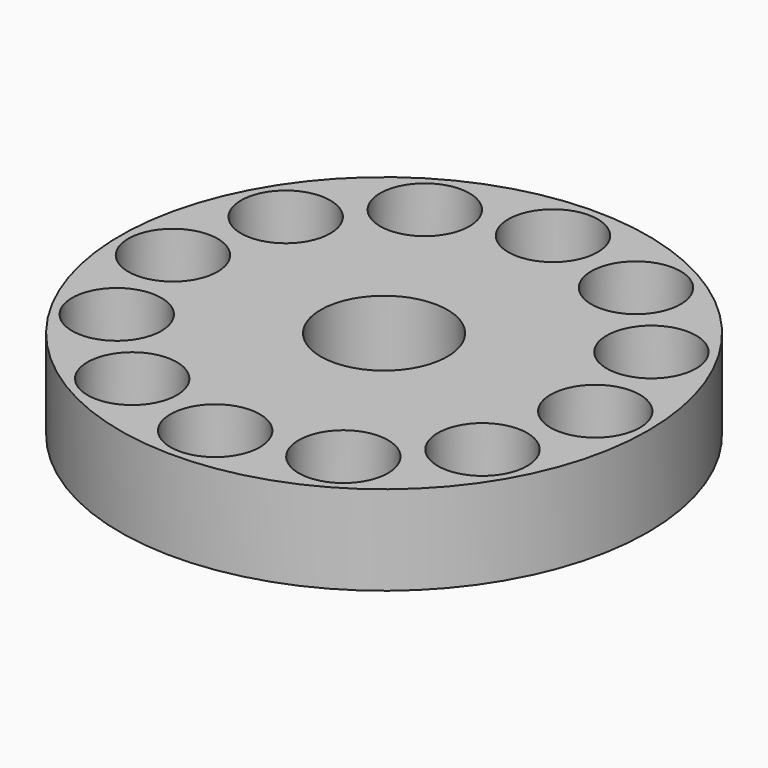
from build123d import *

# Parameters (mm, degrees)
F0_R           = 37.5
F1_DEPTH       = 12.7
F3_D           = 18
F5_D           = 6.5
F5_CBORE_D     = 12.7
F5_CBORE_DEPTH = 10


# Not quite as in the source:
# - a length typed as a fraction of an inch, garbled in the dataset ("3 / 203.2 mm" for 3/8 in), is restored
# - a pattern or mirror of a feature is missing from the dataset's text; its kind, count and spacing are read off the source's solid


with BuildPart() as f1:
    # F0 (on Top) → F1 (new body)
    with BuildSketch(Plane.XY):
        Circle(F0_R)
    extrude(amount=F1_DEPTH)

    # F3 (through all)
    with Locations(Plane.XY.offset(12.7)):
        with Locations((0, 0)):
            Hole(F3_D / 2)

    # F5 (through all)
    with Locations(Plane.XY.offset(12.7)):
        with Locations((0, 30), (25.9807621135, 15), (25.9807621135, -15), (0, -30), (-25.9807621135, -15), (-25.9807621135, 15)):
            f5 = CounterBoreHole(F5_D / 2, F5_CBORE_D / 2, F5_CBORE_DEPTH)

    # F5_copies: F5 across plane
    add(f5.mirror(Plane(origin=(0, 0, 0), x_dir=(-0.7071067812, 0.7071067812, 0), z_dir=(0.7071067812, 0.7071067812, 0))), mode=Mode.SUBTRACT)


solid = f1.part
